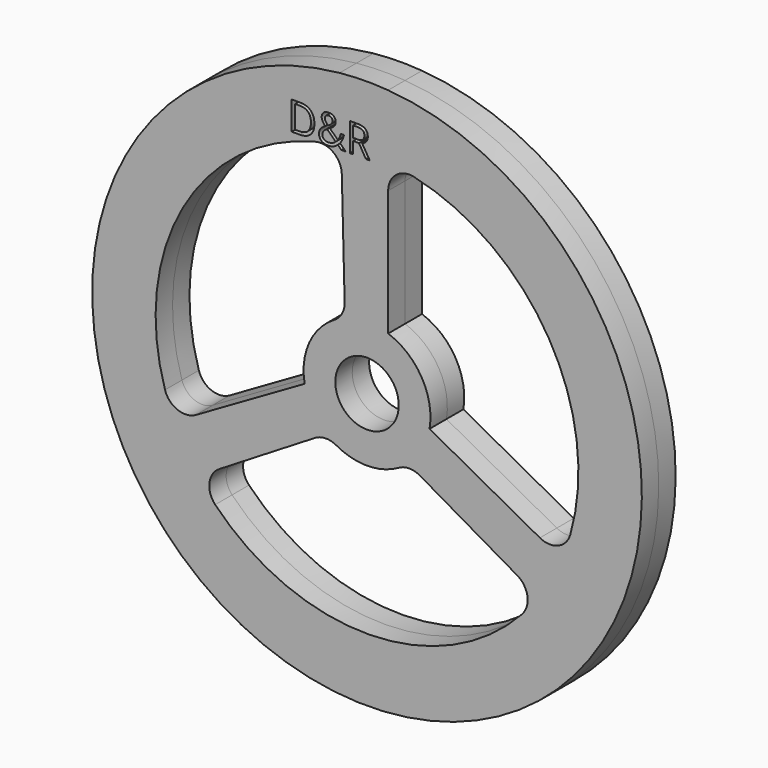
from build123d import *

# Parameters (mm, degrees)
F1_DEPTH     = 1
F2_TEXT_SIZE = 1.8825763623
F3_DEPTH     = 25.4


# Not quite as in the source:
# - Text() gives the source's letters only with a copy of the font that has no kerning and outlines rounded to 1/6400 em; it was checked with that copy


with BuildPart() as f1:
    # F0 (on Front) → F1 (new body, symmetric)
    with BuildSketch(Plane.XZ):
        with BuildLine():
            ThreePointArc((-1.2977340299, 12.9350642205), (-8.7215095486, -9.6402941446), (13, 0))
            ThreePointArc((13, 0), (9.5393920142, 8.8317608663), (1, 12.9614813968))
            ThreePointArc((1, 12.9614813968), (-0.1494518482, 12.9991409003), (-1.2977340299, 12.9350642205))
        make_face()
        with BuildLine():
            ThreePointArc((-7.1816279876, -6.9587512851), (-7.4555144327, -6.137025857), (-6.9851194406, -5.4097191712))
            Line((-6.9851194406, -5.4097191712), (-2.4625183506, -2.6444202546))
            ThreePointArc((-2.4625183506, -2.6444202546), (-1.9619518225, -2.4977996107), (-1.4556480742, -2.62318293))
            ThreePointArc((-1.4556480742, -2.62318293), (0.0254825462, -2.9998917714), (1.5, -2.5980762114))
            ThreePointArc((1.5, -2.5980762114), (2, -2.4641016151), (2.5, -2.5980762114))
            Line((2.5, -2.5980762114), (7.0993420768, -5.2535075975))
            ThreePointArc((7.0993420768, -5.2535075975), (7.5881500594, -5.9703392564), (7.3326023075, -6.7994811125))
            ThreePointArc((7.3326023075, -6.7994811125), (0.1097271994, -9.999397979), (-7.1816279876, -6.9587512851))
        make_face(mode=Mode.SUBTRACT)
        with BuildLine():
            ThreePointArc((-9.5548245298, -2.9504793179), (-8.714596272, 4.9046724473), (-2.4356413977, 9.6988479203))
            ThreePointArc((-2.4356413977, 9.6988479203), (-1.5870630795, 9.5251778255), (-1.1923945093, 8.7541504696))
            Line((-1.1923945093, 8.7541504696), (-1.0588759434, 3.4548135762))
            ThreePointArc((-1.0588759434, 3.4548135762), (-1.1821820052, 2.9479999247), (-1.543919019, 2.5722196762))
            ThreePointArc((-1.543919019, 2.5722196762), (-2.7353092767, 1.2321051745), (-2.9494897428, -0.5481881586))
            Line((-2.9494897428, -0.5481881586), (-8.0993420768, -3.5214567899))
            ThreePointArc((-8.0993420768, -3.5214567899), (-8.9645404949, -3.586361091), (-9.5548245298, -2.9504793179))
        make_face(mode=Mode.SUBTRACT)
        with BuildLine():
            ThreePointArc((1, 1.1180339887), (1.3693063938, 0.6123724357), (1.5, 0))
            ThreePointArc((1.5, 0), (-0.6123724357, -1.3693063938), (-1, 1.1180339887))
            ThreePointArc((-1, 1.1180339887), (0, 1.5), (1, 1.1180339887))
        make_face(mode=Mode.SUBTRACT)
        with BuildLine():
            Line((1, 2.8284271247), (1, 8.7749643874))
            ThreePointArc((1, 8.7749643874), (1.0504807558, 9.0886731774), (1.1968264099, 9.3707094538))
            ThreePointArc((1.1968264099, 9.3707094538), (1.6531081598, 9.7128695272), (2.2222222222, 9.7499604304))
            ThreePointArc((2.2222222222, 9.7499604304), (8.6048690726, 5.0947255316), (9.6172693853, -2.7400966353))
            ThreePointArc((9.6172693853, -2.7400966353), (9.0425775122, -3.3881519685), (8.1775139499, -3.3444312984))
            Line((8.1775139499, -3.3444312984), (2.9574506367, -0.5034736653))
            ThreePointArc((2.9574506367, -0.5034736653), (2.5866473676, 1.5196234389), (1, 2.8284271247))
        make_face(mode=Mode.SUBTRACT)
    extrude(amount=F1_DEPTH, both=True)

    # F2 (on face) → F3 (cut)
    with BuildSketch(Plane.XZ.offset(1)):
        with Locations((-3.7461470347, 9.7499604304)):
            Text('D&R', F2_TEXT_SIZE, font='Open Sans', text_align=(TextAlign.LEFT, TextAlign.BOTTOM))
    extrude(amount=-F3_DEPTH, mode=Mode.SUBTRACT)


solid = f1.part
